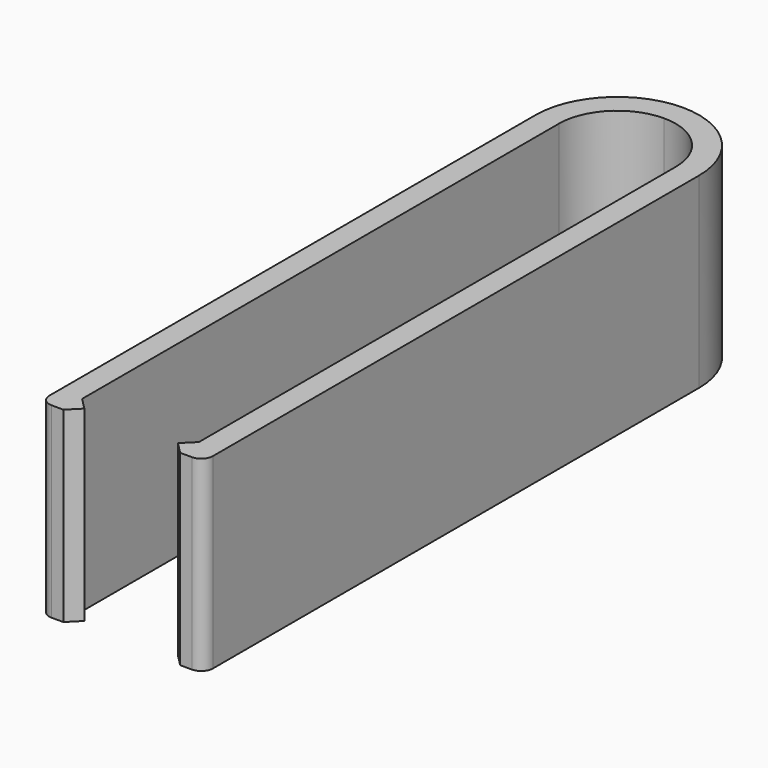
from build123d import *

# Parameters (mm, degrees)
F1_DEPTH = 8
F2_R     = 0.5
F3_SIZE  = 0.49999


# Not quite as in the source:
# - a fillet or chamfer is up to 0.001 mm smaller than in the source, because OpenCascade refuses the exact size


with BuildPart() as f1:
    # F0 (on Top) → F1 (new body)
    with BuildSketch(Plane.XY):
        with BuildLine():
            Line((-2.5, -12.75), (-2.5, 12.75))
            ThreePointArc((-2.5, 12.75), (-1.767766953, 14.517766953), (0, 15.25))
            ThreePointArc((0, 15.25), (1.767766953, 14.517766953), (2.5, 12.75))
            Line((2.5, 12.75), (2.5, -12.75))
            Line((2.5, -12.75), (2, -12.75))
            Line((2, -12.75), (2, -13.75))
            Line((2, -13.75), (3.5, -13.75))
            Line((3.5, -13.75), (3.5, 12.75))
            ThreePointArc((3.5, 12.75), (2.4748737342, 15.2248737342), (0, 16.25))
            ThreePointArc((0, 16.25), (-2.4748737342, 15.2248737342), (-3.5, 12.75))
            Line((-3.5, 12.75), (-3.5, -13.75))
            Line((-3.5, -13.75), (-2, -13.75))
            Line((-2, -13.75), (-2, -12.75))
            Line((-2, -12.75), (-2.5, -12.75))
        make_face()
    extrude(amount=F1_DEPTH)

    # F2
    f2_edges = [f1.edges().sort_by_distance(p)[0] for p in [
        (-3.5, -13.75, 4),
        (3.5, -13.75, 4),
    ]]
    fillet(f2_edges, radius=F2_R)

    # F3 (size 0.5 in the source; OpenCascade refuses exactly that, so slightly less here)
    f3_edges = [f1.edges().sort_by_distance(p)[0] for p in [
        (-2, -13.75, 4),
        (-2, -12.75, 4),
        (2, -13.75, 4),
        (2, -12.75, 4),
    ]]
    chamfer(f3_edges, length=F3_SIZE)


solid = f1.part
